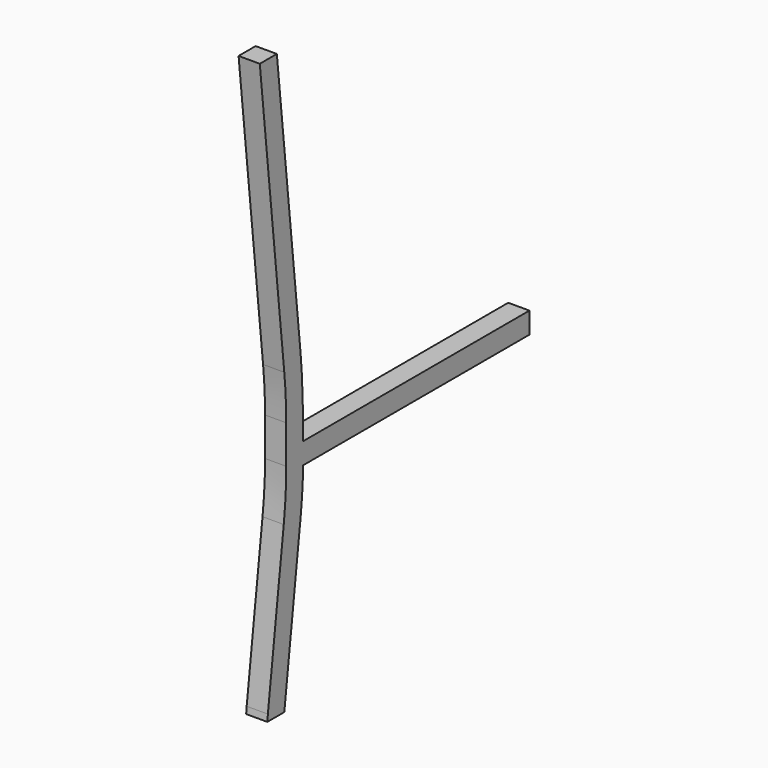
from build123d import *

# Parameters (mm, degrees)
F1_DEPTH    = 30
F2_T1_DEPTH = 163.7053411471
F2_T3_DEPTH = 285.7735535498
F3_T1_DEPTH = 47.177253683
F4_W        = 30
F4_H        = 30
F5_DEPTH    = 400


# Not quite as in the source:
# - a fillet or chamfer that OpenCascade refuses, or shapes differently, is made with other operations: its cross-section is extruded or revolved along the edge and cut away or added


with BuildPart() as f1:
    # F0 (on Right) → F1 (new body)
    with BuildSketch(Plane.YZ):
        with BuildLine():
            Line((0.9376178496, 9.3718236312), (0, 0))
            Line((0, 0), (30, 0))
            Line((30, 0), (58.7747889852, 230.3266173388))
            ThreePointArc((58.7747889852, 230.3266173388), (62.2448009202, 267.4447024247), (63.4029619396, 304.7066385838))
            Line((63.4029619396, 304.7066385838), (63.4029619396, 375))
            Line((63.4029619396, 375), (59.769593104, 426.4305293125))
            Line((59.769593104, 426.4305293125), (16.7944896966, 824.9977231026))
            Line((16.7944896966, 824.9977231026), (16.6203579544, 825))
            Line((16.6203579544, 825), (-13.3796420456, 825))
            Line((-13.3796420456, 825), (29.9452786307, 423.188469929))
            ThreePointArc((29.9452786307, 423.188469929), (32.5379175275, 391.0741192729), (33.4029619396, 358.8668996991))
            Line((33.4029619396, 358.8668996991), (33.4029619396, 304.7066385838))
            ThreePointArc((33.4029619396, 304.7066385838), (32.3027089712, 269.3077992327), (29.0061976329, 234.0456184011))
            Line((29.0061976329, 234.0456184011), (0.9376178496, 9.3718236312))
        make_face()
    extrude(amount=F1_DEPTH)

    # F2: fillet of radius 1450 on 4 edges, made by hand

    # F2_s2 → F2_t1 (cut)
    with BuildSketch(Plane.YZ.offset(-66.8526705736)):
        with BuildLine():
            ThreePointArc((61.6540498994, 399.7559430432), (59.5240083024, 426.4086220464), (56.9028806071, 453.0174939664))
            Line((56.9028806071, 453.0174939664), (59.769593104, 426.4305293125))
            Line((59.769593104, 426.4305293125), (61.6540498994, 399.7559430432))
        make_face()
    extrude(amount=F2_T1_DEPTH, mode=Mode.SUBTRACT)

    # F2_s4 → F2_t3 (cut)
    with BuildSketch(Plane.YZ.offset(-127.8867767749)):
        with BuildLine():
            ThreePointArc((63.4029619396, 323.84528929), (62.5014570183, 374.968195708), (59.7980632353, 426.027533089))
            Line((59.7980632353, 426.027533089), (63.4029619396, 375))
            Line((63.4029619396, 375), (63.4029619396, 323.84528929))
        make_face()
    extrude(amount=F2_T3_DEPTH, mode=Mode.SUBTRACT)

    # F3: fillet of radius 300 on 4 edges, made by hand

    # F3_s2 → F3_t1 (cut)
    with BuildSketch(Plane.YZ.offset(-8.5886268415)):
        with BuildLine():
            ThreePointArc((60.3891403463, 416.3117677563), (60.6508457711, 412.8864247118), (60.8733107804, 409.4583094831))
            ThreePointArc((60.8733107804, 409.4583094831), (60.7708746607, 411.1729780567), (60.666407351, 412.8875240775))
            ThreePointArc((60.666407351, 412.8875240775), (60.5287879715, 414.5997280322), (60.3891403463, 416.3117677563))
        make_face()
    extrude(amount=F3_T1_DEPTH, mode=Mode.SUBTRACT)

    # F4 (on face) → F5 (join)
    with BuildSketch(Plane(origin=(0, 63.4029619396, 0), x_dir=(-1, 0, 0), z_dir=(0, 1, 0))):
        with Locations((-15, 308.84528929)):
            Rectangle(F4_W, F4_H)
    extrude(amount=F5_DEPTH)


solid = f1.part
